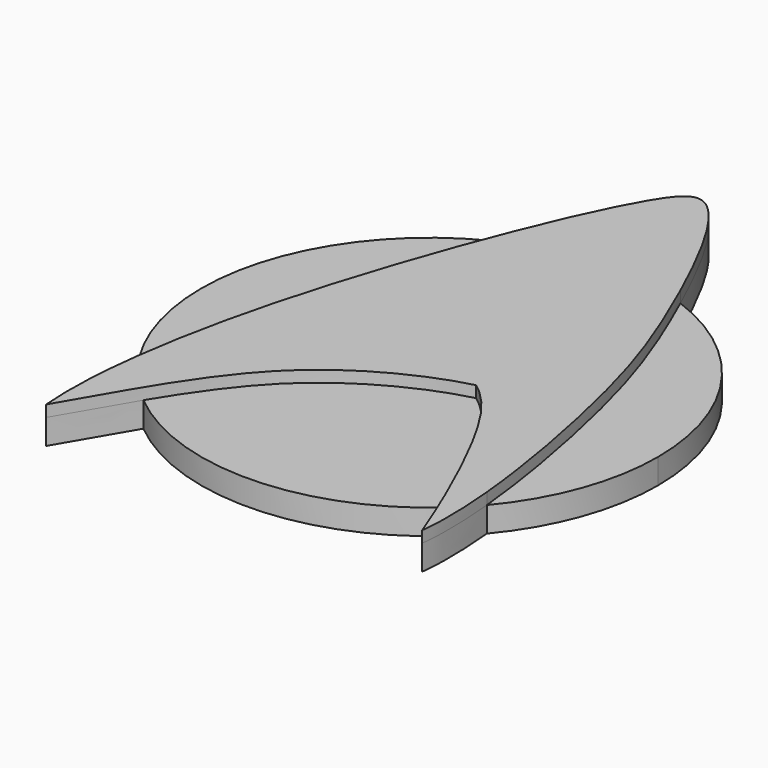
from build123d import *

# Parameters (mm, degrees)
F1_DEPTH = 2.2
F2_DEPTH = 3.2


with BuildPart() as f1:
    # F0 (on Top) → F1 (new body)
    with BuildSketch(Plane.XY):
        with BuildLine():
            ThreePointArc((47.0567276318, 18.8773899614), (50.5400845213, 24.8992537865), (51.75, 31.75))
            ThreePointArc((51.75, 31.75), (48.1739643306, 43.1628609764), (38.7246604334, 50.4944421586))
            add(Edge.make_bspline(
                [(38.7246604334, 50.4944421586), (38.9609346181, 49.9686786288), (41.6774554399, 43.8176291657), (44.2250191929, 36.4340414246), (46.6159564174, 23.5665925252), (47.0567276318, 18.8773899614)],
                knots=[0.630442373, 0.630442373, 0.630442373, 0.630442373, 0.6456439018, 0.8103538291, 0.929794225, 0.929794225, 0.929794225, 0.929794225], degree=3))
        make_face()
        with BuildLine():
            add(Edge.make_bspline(
                [(38.7246604334, 50.4944421586), (38.9609346181, 49.9686786288), (41.6774554399, 43.8176291657), (44.2250191929, 36.4340414246), (46.6159564174, 23.5665925252), (47.0567276318, 18.8773899614)],
                knots=[0.630442373, 0.630442373, 0.630442373, 0.630442373, 0.6456439018, 0.8103538291, 0.929794225, 0.929794225, 0.929794225, 0.929794225], degree=3))
            ThreePointArc((38.7246604334, 50.4944421586), (31.5618373499, 51.7491148508), (24.4238894806, 50.3598926557))
            add(Edge.make_bspline(
                [(15.7865923671, 19.7013645276), (16.2278990367, 23.0877163293), (18.1065072741, 32.7418176771), (22.097534659, 44.5584231861), (24.4238894806, 50.3598926557)],
                knots=[0.0983218299, 0.0983218299, 0.0983218299, 0.0983218299, 0.1865319985, 0.3205820871, 0.3205820871, 0.3205820871, 0.3205820871], degree=3))
            ThreePointArc((15.7865923672, 19.7013645276), (17.2967492534, 17.9259794974), (19.0032017299, 16.3383442206))
            add(Edge.make_bspline(
                [(19.0032017299, 16.3383442206), (20.8233538612, 19.3366897096), (25.818648602, 26.6169979909), (33.4803777859, 30.0196222141), (36.5823023021, 30.7882130146)],
                knots=[0.2222997297, 0.2222997297, 0.2222997297, 0.2222997297, 0.5388931801, 1, 1, 1, 1], degree=3))
            add(Edge.make_bspline(
                [(45.0616821781, 16.8235430329), (44.1054826127, 19.0614489649), (41.7058120017, 24.2306114406), (38.7451071997, 29.2835529549), (36.5823023021, 30.7882130146)],
                knots=[0.2242106798, 0.2242106798, 0.2242106798, 0.2242106798, 0.5365477963, 1, 1, 1, 1], degree=3))
            ThreePointArc((45.0616821781, 16.8235430329), (46.0960069989, 17.8147180442), (47.0567276318, 18.8773899614))
        make_face()
        with BuildLine():
            ThreePointArc((24.4238894806, 50.3598926557), (31.5618373499, 51.7491148508), (38.7246604334, 50.4944421586))
            add(Edge.make_bspline(
                [(24.4238894806, 50.3598926557), (25.9905275085, 54.2667784859), (28.8395118431, 60.4223481909), (32.1998298153, 63.8051247243), (36.5212033159, 55.3976328882), (38.7246604334, 50.4944421586)],
                knots=[0.3205820871, 0.3205820871, 0.3205820871, 0.3205820871, 0.4108554902, 0.4886752267, 0.630442373, 0.630442373, 0.630442373, 0.630442373], degree=3))
        make_face()
        with BuildLine():
            add(Edge.make_bspline(
                [(47.0567276318, 18.8773899614), (47.3158081923, 16.1211273275), (47.379945731, 13.6134596383), (47.1355328849, 11.710731416)],
                knots=[0.929794225, 0.929794225, 0.929794225, 0.929794225, 1, 1, 1, 1], degree=3))
            ThreePointArc((47.0567276318, 18.8773899614), (46.0960069989, 17.8147180442), (45.0616821781, 16.8235430329))
            add(Edge.make_bspline(
                [(47.1355328849, 11.710731416), (46.4293822406, 13.5298032206), (45.7480884465, 15.2170659798), (45.0616821781, 16.8235430329)],
                knots=[0, 0, 0, 0, 0.2242106798, 0.2242106798, 0.2242106798, 0.2242106798], degree=3))
        make_face()
        with BuildLine():
            add(Edge.make_bspline(
                [(15.7865923671, 19.7013645276), (16.2278990367, 23.0877163293), (18.1065072741, 32.7418176771), (22.097534659, 44.5584231861), (24.4238894806, 50.3598926557)],
                knots=[0.0983218299, 0.0983218299, 0.0983218299, 0.0983218299, 0.1865319985, 0.3205820871, 0.3205820871, 0.3205820871, 0.3205820871], degree=3))
            ThreePointArc((24.4238894806, 50.3598926557), (12.4993701223, 37.1733983178), (15.7865923672, 19.7013645276))
        make_face()
        with BuildLine():
            ThreePointArc((19.0032017299, 16.3383442206), (32.1223277175, 11.7534659986), (45.0616821781, 16.8235430329))
            add(Edge.make_bspline(
                [(45.0616821781, 16.8235430329), (44.1054826127, 19.0614489649), (41.7058120017, 24.2306114406), (38.7451071997, 29.2835529549), (36.5823023021, 30.7882130146)],
                knots=[0.2242106798, 0.2242106798, 0.2242106798, 0.2242106798, 0.5365477963, 1, 1, 1, 1], degree=3))
            add(Edge.make_bspline(
                [(19.0032017299, 16.3383442206), (20.8233538612, 19.3366897096), (25.818648602, 26.6169979909), (33.4803777859, 30.0196222141), (36.5823023021, 30.7882130146)],
                knots=[0.2222997297, 0.2222997297, 0.2222997297, 0.2222997297, 0.5388931801, 1, 1, 1, 1], degree=3))
        make_face()
        with BuildLine():
            ThreePointArc((19.0032017299, 16.3383442206), (17.2967492534, 17.9259794974), (15.7865923672, 19.7013645276))
            add(Edge.make_bspline(
                [(15.4055802766, 10.1816686965), (15.180831424, 12.7053480538), (15.2946980654, 15.9268302417), (15.7865923671, 19.7013645276)],
                knots=[0, 0, 0, 0, 0.0983218299, 0.0983218299, 0.0983218299, 0.0983218299], degree=3))
            add(Edge.make_bspline(
                [(15.4055802766, 10.1816686965), (16.5523225946, 12.1106349554), (17.7251609925, 14.2330214765), (19.0032017299, 16.3383442206)],
                knots=[0, 0, 0, 0, 0.2222997297, 0.2222997297, 0.2222997297, 0.2222997297], degree=3))
        make_face()
    extrude(amount=F1_DEPTH)

    # F0 (on Top) → F2 (join)
    with BuildSketch(Plane.XY):
        with BuildLine():
            add(Edge.make_bspline(
                [(38.7246604334, 50.4944421586), (38.9609346181, 49.9686786288), (41.6774554399, 43.8176291657), (44.2250191929, 36.4340414246), (46.6159564174, 23.5665925252), (47.0567276318, 18.8773899614)],
                knots=[0.630442373, 0.630442373, 0.630442373, 0.630442373, 0.6456439018, 0.8103538291, 0.929794225, 0.929794225, 0.929794225, 0.929794225], degree=3))
            ThreePointArc((38.7246604334, 50.4944421586), (31.5618373499, 51.7491148508), (24.4238894806, 50.3598926557))
            add(Edge.make_bspline(
                [(15.7865923671, 19.7013645276), (16.2278990367, 23.0877163293), (18.1065072741, 32.7418176771), (22.097534659, 44.5584231861), (24.4238894806, 50.3598926557)],
                knots=[0.0983218299, 0.0983218299, 0.0983218299, 0.0983218299, 0.1865319985, 0.3205820871, 0.3205820871, 0.3205820871, 0.3205820871], degree=3))
            ThreePointArc((15.7865923672, 19.7013645276), (17.2967492534, 17.9259794974), (19.0032017299, 16.3383442206))
            add(Edge.make_bspline(
                [(19.0032017299, 16.3383442206), (20.8233538612, 19.3366897096), (25.818648602, 26.6169979909), (33.4803777859, 30.0196222141), (36.5823023021, 30.7882130146)],
                knots=[0.2222997297, 0.2222997297, 0.2222997297, 0.2222997297, 0.5388931801, 1, 1, 1, 1], degree=3))
            add(Edge.make_bspline(
                [(45.0616821781, 16.8235430329), (44.1054826127, 19.0614489649), (41.7058120017, 24.2306114406), (38.7451071997, 29.2835529549), (36.5823023021, 30.7882130146)],
                knots=[0.2242106798, 0.2242106798, 0.2242106798, 0.2242106798, 0.5365477963, 1, 1, 1, 1], degree=3))
            ThreePointArc((45.0616821781, 16.8235430329), (46.0960069989, 17.8147180442), (47.0567276318, 18.8773899614))
        make_face()
        with BuildLine():
            ThreePointArc((24.4238894806, 50.3598926557), (31.5618373499, 51.7491148508), (38.7246604334, 50.4944421586))
            add(Edge.make_bspline(
                [(24.4238894806, 50.3598926557), (25.9905275085, 54.2667784859), (28.8395118431, 60.4223481909), (32.1998298153, 63.8051247243), (36.5212033159, 55.3976328882), (38.7246604334, 50.4944421586)],
                knots=[0.3205820871, 0.3205820871, 0.3205820871, 0.3205820871, 0.4108554902, 0.4886752267, 0.630442373, 0.630442373, 0.630442373, 0.630442373], degree=3))
        make_face()
        with BuildLine():
            add(Edge.make_bspline(
                [(47.0567276318, 18.8773899614), (47.3158081923, 16.1211273275), (47.379945731, 13.6134596383), (47.1355328849, 11.710731416)],
                knots=[0.929794225, 0.929794225, 0.929794225, 0.929794225, 1, 1, 1, 1], degree=3))
            ThreePointArc((47.0567276318, 18.8773899614), (46.0960069989, 17.8147180442), (45.0616821781, 16.8235430329))
            add(Edge.make_bspline(
                [(47.1355328849, 11.710731416), (46.4293822406, 13.5298032206), (45.7480884465, 15.2170659798), (45.0616821781, 16.8235430329)],
                knots=[0, 0, 0, 0, 0.2242106798, 0.2242106798, 0.2242106798, 0.2242106798], degree=3))
        make_face()
        with BuildLine():
            ThreePointArc((19.0032017299, 16.3383442206), (17.2967492534, 17.9259794974), (15.7865923672, 19.7013645276))
            add(Edge.make_bspline(
                [(15.4055802766, 10.1816686965), (15.180831424, 12.7053480538), (15.2946980654, 15.9268302417), (15.7865923671, 19.7013645276)],
                knots=[0, 0, 0, 0, 0.0983218299, 0.0983218299, 0.0983218299, 0.0983218299], degree=3))
            add(Edge.make_bspline(
                [(15.4055802766, 10.1816686965), (16.5523225946, 12.1106349554), (17.7251609925, 14.2330214765), (19.0032017299, 16.3383442206)],
                knots=[0, 0, 0, 0, 0.2222997297, 0.2222997297, 0.2222997297, 0.2222997297], degree=3))
        make_face()
    extrude(amount=F2_DEPTH)


solid = f1.part
